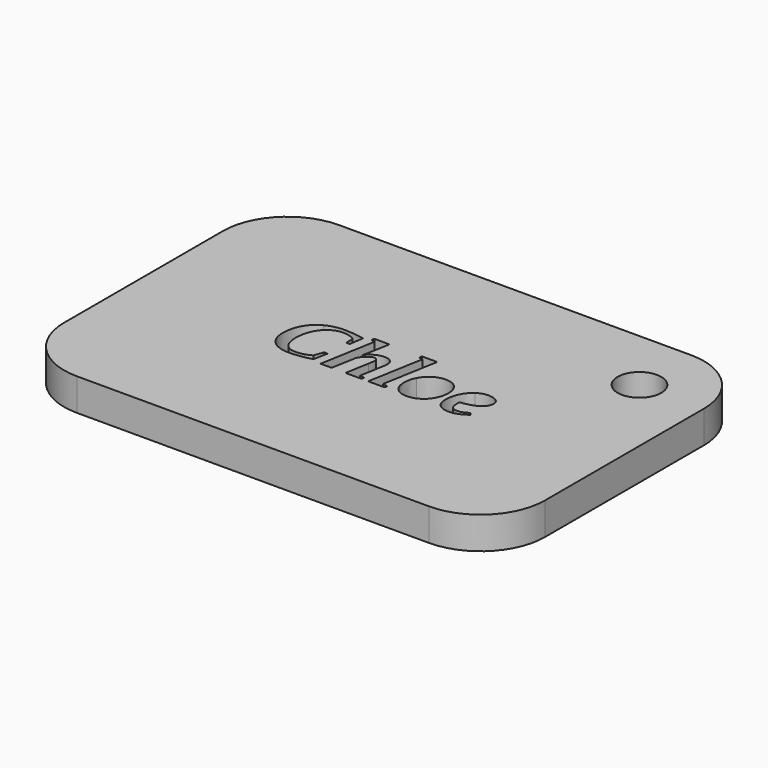
from build123d import *

# Parameters (mm, degrees)
F0_R     = 3.3807298635
F1_DEPTH = 5


with BuildPart() as f1:
    # F0 (on Top) → F1 (new body)
    with BuildSketch(Plane.XY):
        with BuildLine():
            Line((-64.6143609347, 0), (-10, 0))
            ThreePointArc((-10, 0), (-2.9289321881, 2.9289321881), (0, 10))
            Line((0, 10), (0, 40.8130657572))
            ThreePointArc((0, 40.8130657572), (-2.9289321881, 47.8841335691), (-10, 50.8130657572))
            Line((-10, 50.8130657572), (-64.6143609347, 50.8130657572))
            ThreePointArc((-64.6143609347, 50.8130657572), (-71.6854287466, 47.8841335691), (-74.6143609347, 40.8130657572))
            Line((-74.6143609347, 40.8130657572), (-74.6143609347, 10))
            ThreePointArc((-74.6143609347, 10), (-71.6854287466, 2.9289321881), (-64.6143609347, 0))
        make_face()
        with BuildLine():
            add(Edge.make_bspline(
                [(-46.661470066, 21.0336615097), (-47.5455431911, 20.8818405408), (-48.3841733051, 20.8818405408)],
                knots=[0, 0, 0, 1, 1, 1], degree=2))
            add(Edge.make_bspline(
                [(-48.3841733051, 20.8818405408), (-50.2246152549, 20.8818405408), (-51.2408862305, 21.8340781826)],
                knots=[0, 0, 0, 1, 1, 1], degree=2))
            add(Edge.make_bspline(
                [(-51.2408862305, 21.8340781826), (-52.2571572061, 22.7863158244), (-52.2571572061, 24.4387889555)],
                knots=[0, 0, 0, 1, 1, 1], degree=2))
            add(Edge.make_bspline(
                [(-52.2571572061, 24.4387889555), (-52.2571572061, 26.0272287528), (-51.5858399966, 27.2376653213)],
                knots=[0, 0, 0, 1, 1, 1], degree=2))
            add(Edge.make_bspline(
                [(-51.5858399966, 27.2376653213), (-50.9145227871, 28.4481018898), (-49.6689711646, 29.1070255508)],
                knots=[0, 0, 0, 1, 1, 1], degree=2))
            add(Edge.make_bspline(
                [(-49.6689711646, 29.1070255508), (-48.423419542, 29.7659492119), (-46.8225861963, 29.7659492119)],
                knots=[0, 0, 0, 1, 1, 1], degree=2))
            add(Edge.make_bspline(
                [(-46.8225861963, 29.7659492119), (-45.3642786581, 29.7659492119), (-43.7696420866, 29.4292578114)],
                knots=[0, 0, 0, 1, 1, 1], degree=2))
            Line((-43.7696420866, 29.4292578114), (-44.1104646699, 27.2541900526))
            Line((-44.1104646699, 27.2541900526), (-44.6537152117, 27.2541900526))
            Line((-44.6537152117, 27.2541900526), (-44.6537152117, 28.5059384494))
            add(Edge.make_bspline(
                [(-44.6537152117, 28.5059384494), (-45.0028001606, 28.7847932903), (-45.4964765086, 28.9355814635)],
                knots=[0, 0, 0, 1, 1, 1], degree=2))
            add(Edge.make_bspline(
                [(-45.4964765086, 28.9355814635), (-45.9901528565, 29.0863696367), (-46.5313378069, 29.0863696367)],
                knots=[0, 0, 0, 1, 1, 1], degree=2))
            add(Edge.make_bspline(
                [(-46.5313378069, 29.0863696367), (-47.5971829765, 29.0863696367), (-48.4461410476, 28.4925121052)],
                knots=[0, 0, 0, 1, 1, 1], degree=2))
            add(Edge.make_bspline(
                [(-48.4461410476, 28.4925121052), (-49.2950991187, 27.8986545737), (-49.766053961, 26.8183502643)],
                knots=[0, 0, 0, 1, 1, 1], degree=2))
            add(Edge.make_bspline(
                [(-49.766053961, 26.8183502643), (-50.2370088034, 25.7380459548), (-50.2370088034, 24.3809523959)],
                knots=[0, 0, 0, 1, 1, 1], degree=2))
            add(Edge.make_bspline(
                [(-50.2370088034, 24.3809523959), (-50.2370088034, 23.0445147511), (-49.6431512719, 22.2957378636)],
                knots=[0, 0, 0, 1, 1, 1], degree=2))
            add(Edge.make_bspline(
                [(-49.6431512719, 22.2957378636), (-49.0492937404, 21.5469609761), (-47.9710550224, 21.5469609761)],
                knots=[0, 0, 0, 1, 1, 1], degree=2))
            add(Edge.make_bspline(
                [(-47.9710550224, 21.5469609761), (-47.3389840497, 21.5469609761), (-46.6996835071, 21.7318314076)],
                knots=[0, 0, 0, 1, 1, 1], degree=2))
            add(Edge.make_bspline(
                [(-46.6996835071, 21.7318314076), (-46.0603829645, 21.9167018392), (-45.6679205959, 22.1996878629)],
                knots=[0, 0, 0, 1, 1, 1], degree=2))
            Line((-45.6679205959, 22.1996878629), (-45.1701130652, 23.6208147556))
            Line((-45.1701130652, 23.6208147556), (-44.6206657491, 23.6208147556))
            Line((-44.6206657491, 23.6208147556), (-45.0482431718, 21.4250910827))
            add(Edge.make_bspline(
                [(-45.0482431718, 21.4250910827), (-45.7773969408, 21.1854824787), (-46.661470066, 21.0336615097)],
                knots=[0, 0, 0, 1, 1, 1], degree=2))
        make_face(mode=Mode.SUBTRACT)
        with BuildLine():
            add(Edge.make_bspline(
                [(-28.4233306773, 21.3889432329), (-29.2340753072, 20.8818405408), (-30.2462151, 20.8818405408)],
                knots=[0, 0, 0, 1, 1, 1], degree=2))
            add(Edge.make_bspline(
                [(-30.2462151, 20.8818405408), (-31.3430441408, 20.8818405408), (-32.0019678018, 21.5727808688)],
                knots=[0, 0, 0, 1, 1, 1], degree=2))
            add(Edge.make_bspline(
                [(-32.0019678018, 21.5727808688), (-32.6608914628, 22.2637211967), (-32.6608914628, 23.4266491627)],
                knots=[0, 0, 0, 1, 1, 1], degree=2))
            add(Edge.make_bspline(
                [(-32.6608914628, 23.4266491627), (-32.6608914628, 24.4718384181), (-32.2085269432, 25.349714769)],
                knots=[0, 0, 0, 1, 1, 1], degree=2))
            add(Edge.make_bspline(
                [(-32.2085269432, 25.349714769), (-31.7561624235, 26.2275911199), (-30.9464505893, 26.734693812)],
                knots=[0, 0, 0, 1, 1, 1], degree=2))
            add(Edge.make_bspline(
                [(-30.9464505893, 26.734693812), (-30.1367387551, 27.2417965041), (-29.1225333709, 27.2417965041)],
                knots=[0, 0, 0, 1, 1, 1], degree=2))
            add(Edge.make_bspline(
                [(-29.1225333709, 27.2417965041), (-28.0257043301, 27.2417965041), (-27.3678134648, 26.5508561762)],
                knots=[0, 0, 0, 1, 1, 1], degree=2))
            add(Edge.make_bspline(
                [(-27.3678134648, 26.5508561762), (-26.7099225995, 25.8599158482), (-26.7099225995, 24.6969878822)],
                knots=[0, 0, 0, 1, 1, 1], degree=2))
            add(Edge.make_bspline(
                [(-26.7099225995, 24.6969878822), (-26.7099225995, 23.6517986268), (-27.1612543234, 22.7739222759)],
                knots=[0, 0, 0, 1, 1, 1], degree=2))
            add(Edge.make_bspline(
                [(-27.1612543234, 22.7739222759), (-27.6125860473, 21.896045925), (-28.4233306773, 21.3889432329)],
                knots=[0, 0, 0, 1, 1, 1], degree=2))
        make_face(mode=Mode.SUBTRACT)
        with BuildLine():
            add(Edge.make_bspline(
                [(-21.2061542772, 26.8834163938), (-20.6804612624, 26.5250362835), (-20.6804612624, 25.9177524078)],
                knots=[0, 0, 0, 1, 1, 1], degree=2))
            add(Edge.make_bspline(
                [(-20.6804612624, 25.9177524078), (-20.6804612624, 25.3373212205), (-21.1059730937, 24.8467432597)],
                knots=[0, 0, 0, 1, 1, 1], degree=2))
            add(Edge.make_bspline(
                [(-21.1059730937, 24.8467432597), (-21.5314849249, 24.3561652989), (-22.3360327806, 24.0401298126)],
                knots=[0, 0, 0, 1, 1, 1], degree=2))
            add(Edge.make_bspline(
                [(-22.3360327806, 24.0401298126), (-23.1405806363, 23.7240943263), (-24.1589172033, 23.6456018526)],
                knots=[0, 0, 0, 1, 1, 1], degree=2))
            add(Edge.make_bspline(
                [(-24.1589172033, 23.6456018526), (-24.191966666, 23.5175351849), (-24.191966666, 23.2076964728)],
                knots=[0, 0, 0, 1, 1, 1], degree=2))
            add(Edge.make_bspline(
                [(-24.191966666, 23.2076964728), (-24.191966666, 21.6832900094), (-23.0228419257, 21.6832900094)],
                knots=[0, 0, 0, 1, 1, 1], degree=2))
            add(Edge.make_bspline(
                [(-23.0228419257, 21.6832900094), (-22.5456903091, 21.6832900094), (-22.1387688006, 21.8671276452)],
                knots=[0, 0, 0, 1, 1, 1], degree=2))
            add(Edge.make_bspline(
                [(-22.1387688006, 21.8671276452), (-21.7318472921, 22.0509652811), (-21.3765655689, 22.2905738851)],
                knots=[0, 0, 0, 1, 1, 1], degree=2))
            Line((-21.3765655689, 22.2905738851), (-21.0935795452, 21.8836523765))
            add(Edge.make_bspline(
                [(-21.0935795452, 21.8836523765), (-21.661617184, 21.4065007599), (-22.3267376192, 21.1441706504)],
                knots=[0, 0, 0, 1, 1, 1], degree=2))
            add(Edge.make_bspline(
                [(-22.3267376192, 21.1441706504), (-22.9918580545, 20.8818405408), (-23.6053387044, 20.8818405408)],
                knots=[0, 0, 0, 1, 1, 1], degree=2))
            add(Edge.make_bspline(
                [(-23.6053387044, 20.8818405408), (-24.7476107563, 20.8818405408), (-25.347665062, 21.4571077496)],
                knots=[0, 0, 0, 1, 1, 1], degree=2))
            add(Edge.make_bspline(
                [(-25.347665062, 21.4571077496), (-25.9477193678, 22.0323749583), (-25.9477193678, 23.1426303433)],
                knots=[0, 0, 0, 1, 1, 1], degree=2))
            add(Edge.make_bspline(
                [(-25.9477193678, 23.1426303433), (-25.9477193678, 24.2528857282), (-25.4767645254, 25.2020249829)],
                knots=[0, 0, 0, 1, 1, 1], degree=2))
            add(Edge.make_bspline(
                [(-25.4767645254, 25.2020249829), (-25.005809683, 26.1511642376), (-24.2312129028, 26.6964803709)],
                knots=[0, 0, 0, 1, 1, 1], degree=2))
            add(Edge.make_bspline(
                [(-24.2312129028, 26.6964803709), (-23.4566161226, 27.2417965041), (-22.6241827828, 27.2417965041)],
                knots=[0, 0, 0, 1, 1, 1], degree=2))
            add(Edge.make_bspline(
                [(-22.6241827828, 27.2417965041), (-21.7318472921, 27.2417965041), (-21.2061542772, 26.8834163938)],
                knots=[0, 0, 0, 1, 1, 1], degree=2))
        make_face(mode=Mode.SUBTRACT)
        with BuildLine():
            Line((-41.0327334632, 26.1635577861), (-41.0761108829, 25.9755889674))
            add(Edge.make_bspline(
                [(-41.0761108829, 25.9755889674), (-40.0825614128, 27.2417965041), (-38.6118603262, 27.2417965041)],
                knots=[0, 0, 0, 1, 1, 1], degree=2))
            add(Edge.make_bspline(
                [(-38.6118603262, 27.2417965041), (-37.9859861278, 27.2417965041), (-37.6048845119, 26.8958099423)],
                knots=[0, 0, 0, 1, 1, 1], degree=2))
            add(Edge.make_bspline(
                [(-37.6048845119, 26.8958099423), (-37.223782896, 26.5498233805), (-37.223782896, 25.9569986447)],
                knots=[0, 0, 0, 1, 1, 1], degree=2))
            add(Edge.make_bspline(
                [(-37.223782896, 25.9569986447), (-37.223782896, 25.6203072442), (-37.333259241, 25.0212857342)],
                knots=[0, 0, 0, 1, 1, 1], degree=2))
            Line((-37.333259241, 25.0212857342), (-37.9467398909, 21.5924039872))
            Line((-37.9467398909, 21.5924039872), (-37.1969302077, 21.4374846312))
            Line((-37.1969302077, 21.4374846312), (-37.2816194556, 21.0119727999))
            Line((-37.2816194556, 21.0119727999), (-39.7727227007, 21.0119727999))
            Line((-39.7727227007, 21.0119727999), (-39.1137990397, 24.6845943337))
            add(Edge.make_bspline(
                [(-39.1137990397, 24.6845943337), (-38.9733388236, 25.434404017), (-38.9733388236, 25.6926029437)],
                knots=[0, 0, 0, 1, 1, 1], degree=2))
            add(Edge.make_bspline(
                [(-38.9733388236, 25.6926029437), (-38.9733388236, 26.3184771421), (-39.5599667851, 26.3184771421)],
                knots=[0, 0, 0, 1, 1, 1], degree=2))
            add(Edge.make_bspline(
                [(-39.5599667851, 26.3184771421), (-39.9668882936, 26.3184771421), (-40.4770893729, 25.8661126225)],
                knots=[0, 0, 0, 1, 1, 1], degree=2))
            add(Edge.make_bspline(
                [(-40.4770893729, 25.8661126225), (-40.9872904521, 25.4137481028), (-41.2310302389, 24.845710464)],
                knots=[0, 0, 0, 1, 1, 1], degree=2))
            Line((-41.2310302389, 24.845710464), (-41.9168065883, 21.0119727999))
            Line((-41.9168065883, 21.0119727999), (-43.6333130533, 21.0119727999))
            Line((-43.6333130533, 21.0119727999), (-42.1233657297, 29.6027674902))
            Line((-42.1233657297, 29.6027674902), (-42.7099936913, 29.7576868462))
            Line((-42.7099936913, 29.7576868462), (-42.6397635832, 30.1852642689))
            Line((-42.6397635832, 30.1852642689), (-40.28292378, 30.1852642689))
            Line((-40.28292378, 30.1852642689), (-40.8261743218, 27.196353493))
            Line((-40.8261743218, 27.196353493), (-41.0327334632, 26.1635577861))
        make_face(mode=Mode.SUBTRACT)
        Polygon((-32.8860409269, 30.1852642689), (-34.4104473904, 21.5924039872), (-33.6420473844, 21.4374846312), (-33.7122774925, 21.0119727999), (-36.2488237487, 21.0119727999), (-34.7264828767, 29.6027674902), (-35.3131108382, 29.7576868462), (-35.2428807301, 30.1852642689), align=None, mode=Mode.SUBTRACT)
        with Locations((-10, 40.8130657572)):
            Circle(F0_R, mode=Mode.SUBTRACT)
    extrude(amount=F1_DEPTH)


solid = f1.part
